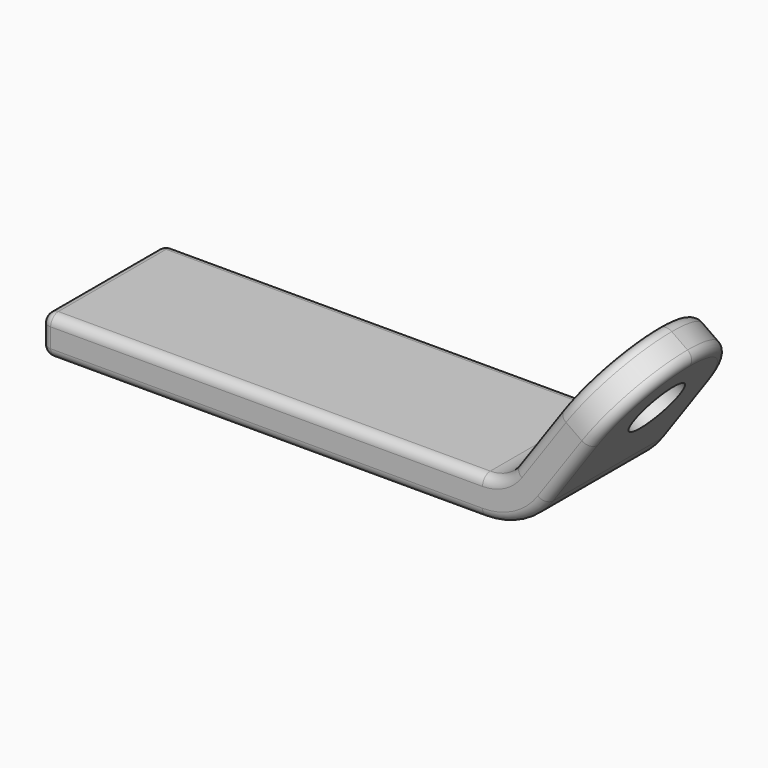
from build123d import *

# Parameters (mm, degrees)
F1_DEPTH     = 25.4
F2_R         = 9.525
F3_DEPTH     = 42.7816898715
F4_R         = 25.39999
F5_R         = 3.175
F6_W         = 5.0767767243
F6_H         = 5.0767767243
F7_DEPTH     = 3.175
F8_T1_DEPTH  = 142.613798458
F8_T3_DEPTH  = 25.40001
F8_T5_DEPTH  = 44.45
F8_T7_DEPTH  = 25.40001
F8_T9_DEPTH  = 2e-05
F8_T12_ANGLE = 90
F8_T14_ANGLE = 55
F8_T16_ANGLE = 55
F8_T18_ANGLE = 90
F8_T20_ANGLE = 90
F8_T22_ANGLE = 90
F8_T24_ANGLE = 55
F8_T26_ANGLE = 90
F8_T28_ANGLE = 90
F8_T30_ANGLE = 90
F8_T32_ANGLE = 55
F8_T34_ANGLE = 90


# Not quite as in the source:
# - a fillet or chamfer that OpenCascade refuses, or shapes differently, is made with other operations: its cross-section is extruded or revolved along the edge and cut away or added
# - a fillet or chamfer is up to 0.001 mm smaller than in the source, because OpenCascade refuses the exact size


with BuildPart() as f1:
    # F0 (on Front) → F1 (new body, symmetric)
    with BuildSketch(Plane.XZ):
        with BuildLine():
            Line((118.9895820573, 10.6313137069), (-26.7992164007, 10.6313137069))
            Line((-26.7992164007, 10.6313137069), (-26.7992164007, -2.0686862931))
            Line((-26.7992164007, -2.0686862931), (118.9895820573, -2.0686862931))
            ThreePointArc((118.9895820573, -2.0686862931), (130.7179968335, 0.8012385441), (139.7960439822, 8.7624722235))
            Line((139.7960439822, 8.7624722235), (168.9337269489, 50.3753960734))
            Line((168.9337269489, 50.3753960734), (158.5304959864, 57.6598168151))
            Line((158.5304959864, 57.6598168151), (129.3928130198, 16.0468929652))
            ThreePointArc((129.3928130198, 16.0468929652), (124.8537894454, 12.0662761255), (118.9895820573, 10.6313137069))
        make_face()
    extrude(amount=F1_DEPTH, both=True)

    # F2 (on face) → F3 (cut, through all)
    with BuildSketch(Plane(origin=(79.2843072841, 0, -55.515469622), x_dir=(0, -1, 0), z_dir=(-0.8191520443, 0, 0.5735764364))):
        with Locations((0, 115.9365137582)):
            Circle(F2_R)
    extrude(amount=-F3_DEPTH, mode=Mode.SUBTRACT)

    # F4 (radius 25.4 in the source; OpenCascade refuses exactly that, so slightly less here)
    f4_edges = [f1.edges().sort_by_distance(p)[0] for p in [
        (163.732111, 25.4, 54.017606),
        (163.732111, -25.4, 54.017606),
    ]]
    fillet(f4_edges, radius=F4_R)

    # F5
    f5_edges = [f1.edges().sort_by_distance(p)[0] for p in [
        (-26.799216, -25.4, 4.281314),
        (-26.799216, 25.4, 4.281314),
    ]]
    fillet(f5_edges, radius=F5_R)

    # F6 (on face) → F7 (cut)
    with BuildSketch(Plane(origin=(0, 0, -2.0686862931), x_dir=(1, 0, 0), z_dir=(0, 0, -1))):
        with Locations((4.9507835993, 0)):
            Rectangle(F6_W, F6_H)
    extrude(amount=-F7_DEPTH, mode=Mode.SUBTRACT)

    # F8: fillet of radius 3.175 on 24 edges, made by hand

    # F8_s2 → F8_t1 (cut)
    with BuildSketch(Plane.YZ.offset(-23.6242164007)):
        with BuildLine():
            ThreePointArc((25.4, 7.4563137069), (24.4700640303, 9.7013777371), (22.225, 10.6313137069))
            Line((22.225, 10.6313137069), (25.4, 10.6313137069))
            Line((25.4, 10.6313137069), (25.4, 7.4563137069))
        make_face()
        with BuildLine():
            ThreePointArc((-22.225, 10.6313137069), (-24.4700640303, 9.7013777371), (-25.4, 7.4563137069))
            Line((-25.4, 7.4563137069), (-25.4, 10.6313137069))
            Line((-25.4, 10.6313137069), (-22.225, 10.6313137069))
        make_face()
        with BuildLine():
            ThreePointArc((-22.225, -2.0686862931), (-24.4700640303, -1.1387503234), (-25.4, 1.1063137069))
            Line((-25.4, 1.1063137069), (-25.4, -2.0686862931))
            Line((-25.4, -2.0686862931), (-22.225, -2.0686862931))
        make_face()
        with BuildLine():
            ThreePointArc((25.4, 1.1063137069), (24.4700640303, -1.1387503234), (22.225, -2.0686862931))
            Line((22.225, -2.0686862931), (25.4, -2.0686862931))
            Line((25.4, -2.0686862931), (25.4, 1.1063137069))
        make_face()
    extrude(amount=F8_T1_DEPTH, mode=Mode.SUBTRACT)

    # F8_s4 → F8_t3 (cut)
    with BuildSketch(Plane(origin=(64.6773529548, 0, 92.3688327037), x_dir=(0, 1, 0), z_dir=(-0.5735764364, 0, -0.8191520443))):
        with BuildLine():
            ThreePointArc((25.4, 99.96326762), (24.4700640303, 97.7182035897), (22.225, 96.78826762))
            Line((22.225, 96.78826762), (25.4, 96.78826762))
            Line((25.4, 96.78826762), (25.4, 99.96326762))
        make_face()
        with BuildLine():
            ThreePointArc((-22.225, 96.78826762), (-24.4700640303, 97.7182035897), (-25.4, 99.96326762))
            Line((-25.4, 99.96326762), (-25.4, 96.78826762))
            Line((-25.4, 96.78826762), (-22.225, 96.78826762))
        make_face()
    extrude(amount=F8_T3_DEPTH, mode=Mode.SUBTRACT)

    # F8_s6 → F8_t5 (cut)
    with BuildSketch(Plane.XZ.offset(-22.225)):
        with BuildLine():
            ThreePointArc((-23.6242164007, 10.6313137069), (-25.869280431, 9.7013777371), (-26.7992164007, 7.4563137069))
            Line((-26.7992164007, 7.4563137069), (-26.7992164007, 10.6313137069))
            Line((-26.7992164007, 10.6313137069), (-23.6242164007, 10.6313137069))
        make_face()
        with BuildLine():
            ThreePointArc((-23.6242164007, -2.0686862931), (-25.869280431, -1.1387503234), (-26.7992164007, 1.1063137069))
            Line((-26.7992164007, 1.1063137069), (-26.7992164007, -2.0686862931))
            Line((-26.7992164007, -2.0686862931), (-23.6242164007, -2.0686862931))
        make_face()
    extrude(amount=F8_T5_DEPTH, mode=Mode.SUBTRACT)

    # F8_s8 → F8_t7 (cut)
    with BuildSketch(Plane(origin=(50.1085057357, 0, 71.5623625873), x_dir=(0, 1, 0), z_dir=(0.5735764364, 0, 0.8191520443))):
        with BuildLine():
            ThreePointArc((25.4, -106.31326762), (24.4700640303, -108.5583316502), (22.225, -109.48826762))
            Line((22.225, -109.48826762), (25.4, -109.48826762))
            Line((25.4, -109.48826762), (25.4, -106.31326762))
        make_face()
        with BuildLine():
            ThreePointArc((-22.225, -109.48826762), (-24.4700640303, -108.5583316502), (-25.4, -106.31326762))
            Line((-25.4, -106.31326762), (-25.4, -109.48826762))
            Line((-25.4, -109.48826762), (-22.225, -109.48826762))
        make_face()
    extrude(amount=F8_T7_DEPTH, mode=Mode.SUBTRACT)

    # F8_s10 → F8_t9 (cut)
    with BuildSketch(Plane.XZ.offset(-1e-05)):
        with BuildLine():
            ThreePointArc((167.1126217635, 47.7745883328), (167.6385786386, 50.1470264823), (166.3329192083, 52.1965012588))
            Line((166.3329192083, 52.1965012588), (168.9337269489, 50.3753960734))
            Line((168.9337269489, 50.3753960734), (167.1126217635, 47.7745883328))
        make_face()
        with BuildLine():
            ThreePointArc((156.709390801, 55.0590090745), (158.7588655775, 56.3646685049), (161.131303727, 55.8387116297))
            Line((161.131303727, 55.8387116297), (158.5304959864, 57.6598168151))
            Line((158.5304959864, 57.6598168151), (156.709390801, 55.0590090745))
        make_face()
    extrude(amount=F8_T9_DEPTH, mode=Mode.SUBTRACT)

    # F8_s11 → F8_t12 (revolve, cut)
    with BuildSketch(Plane(origin=(64.6773529548, 0, 92.3688327037), x_dir=(0, 1, 0), z_dir=(-0.5735764364, 0, -0.8191520443))):
        with BuildLine():
            ThreePointArc((25.4, 99.96326762), (24.4700640303, 97.7182035897), (22.225, 96.78826762))
            Line((22.225, 96.78826762), (25.4, 96.78826762))
            Line((25.4, 96.78826762), (25.4, 99.96326762))
        make_face()
    revolve(axis=Axis((143.9616602388, 1e-05, 36.8533630817), (0.8191520443, 0, -0.5735764364)), revolution_arc=F8_T12_ANGLE, mode=Mode.SUBTRACT)

    # F8_s13 → F8_t14 (revolve, cut)
    with BuildSketch(Plane.YZ.offset(118.9895820573)):
        with BuildLine():
            ThreePointArc((25.4, 1.1063137069), (24.4700640303, -1.1387503234), (22.225, -2.0686862931))
            Line((22.225, -2.0686862931), (25.4, -2.0686862931))
            Line((25.4, -2.0686862931), (25.4, 1.1063137069))
        make_face()
    revolve(axis=Axis((118.9895820573, 25.4, 23.3313137069), (0, -1, 0)), revolution_arc=F8_T14_ANGLE, mode=Mode.SUBTRACT)

    # F8_s15 → F8_t16 (revolve, cut)
    with BuildSketch(Plane(origin=(50.1085057357, 0, 71.5623625873), x_dir=(0, 1, 0), z_dir=(0.5735764364, 0, 0.8191520443))):
        with BuildLine():
            ThreePointArc((25.4, -99.96326762), (24.4700640303, -97.7182035897), (22.225, -96.78826762))
            Line((22.225, -96.78826762), (25.4, -96.78826762))
            Line((25.4, -96.78826762), (25.4, -99.96326762))
        make_face()
    revolve(axis=Axis((118.9895820573, 25.4, 23.3313137069), (0, 1, 0)), revolution_arc=F8_T16_ANGLE, mode=Mode.SUBTRACT)

    # F8_s17 → F8_t18 (revolve, cut)
    with BuildSketch(Plane.YZ.offset(-23.6242164007)):
        with BuildLine():
            ThreePointArc((22.225, -2.0686862931), (24.4700640303, -1.1387503234), (25.4, 1.1063137069))
            Line((25.4, 1.1063137069), (25.4, -2.0686862931))
            Line((25.4, -2.0686862931), (22.225, -2.0686862931))
        make_face()
    revolve(axis=Axis((-23.6242164007, 22.225, -2.0686862931), (0, 0, 1)), revolution_arc=F8_T18_ANGLE, mode=Mode.SUBTRACT)

    # F8_s19 → F8_t20 (revolve, cut)
    with BuildSketch(Plane.YZ.offset(-23.6242164007)):
        with BuildLine():
            ThreePointArc((-22.225, -2.0686862931), (-24.4700640303, -1.1387503234), (-25.4, 1.1063137069))
            Line((-25.4, 1.1063137069), (-25.4, -2.0686862931))
            Line((-25.4, -2.0686862931), (-22.225, -2.0686862931))
        make_face()
    revolve(axis=Axis((-23.6242164007, -22.225, -2.0686862931), (0, 0, -1)), revolution_arc=F8_T20_ANGLE, mode=Mode.SUBTRACT)

    # F8_s21 → F8_t22 (revolve, cut)
    with BuildSketch(Plane.YZ.offset(-23.6242164007)):
        with BuildLine():
            ThreePointArc((25.4, 7.4563137069), (24.4700640303, 9.7013777371), (22.225, 10.6313137069))
            Line((22.225, 10.6313137069), (25.4, 10.6313137069))
            Line((25.4, 10.6313137069), (25.4, 7.4563137069))
        make_face()
    revolve(axis=Axis((-23.6242164007, 22.225, 10.6313137069), (0, 0, 1)), revolution_arc=F8_T22_ANGLE, mode=Mode.SUBTRACT)

    # F8_s23 → F8_t24 (revolve, cut)
    with BuildSketch(Plane.YZ.offset(118.9895820573)):
        with BuildLine():
            ThreePointArc((-22.225, -2.0686862931), (-24.4700640303, -1.1387503234), (-25.4, 1.1063137069))
            Line((-25.4, 1.1063137069), (-25.4, -2.0686862931))
            Line((-25.4, -2.0686862931), (-22.225, -2.0686862931))
        make_face()
    revolve(axis=Axis((118.9895820573, -25.4, 23.3313137069), (0, -1, 0)), revolution_arc=F8_T24_ANGLE, mode=Mode.SUBTRACT)

    # F8_s25 → F8_t26 (revolve, cut)
    with BuildSketch(Plane.YZ.offset(-23.6242164007)):
        with BuildLine():
            ThreePointArc((-22.225, 10.6313137069), (-24.4700640303, 9.7013777371), (-25.4, 7.4563137069))
            Line((-25.4, 7.4563137069), (-25.4, 10.6313137069))
            Line((-25.4, 10.6313137069), (-22.225, 10.6313137069))
        make_face()
    revolve(axis=Axis((-23.6242164007, -22.225, 10.6313137069), (0, 0, -1)), revolution_arc=F8_T26_ANGLE, mode=Mode.SUBTRACT)

    # F8_s27 → F8_t28 (revolve, cut)
    with BuildSketch(Plane(origin=(64.6773529548, 0, 92.3688327037), x_dir=(0, 1, 0), z_dir=(-0.5735764364, 0, -0.8191520443))):
        with BuildLine():
            ThreePointArc((22.225, 109.48826762), (24.4700640303, 108.5583316502), (25.4, 106.31326762))
            Line((25.4, 106.31326762), (25.4, 109.48826762))
            Line((25.4, 109.48826762), (22.225, 109.48826762))
        make_face()
    revolve(axis=Axis((154.3648912013, 1e-05, 29.56894234), (0.8191520443, 0, -0.5735764364)), revolution_arc=F8_T28_ANGLE, mode=Mode.SUBTRACT)

    # F8_s29 → F8_t30 (revolve, cut)
    with BuildSketch(Plane.XZ.offset(1e-05)):
        with BuildLine():
            ThreePointArc((167.1126217635, 47.7745883328), (167.6385786386, 50.1470264823), (166.3329192083, 52.1965012588))
            Line((166.3329192083, 52.1965012588), (168.9337269489, 50.3753960734))
            Line((168.9337269489, 50.3753960734), (167.1126217635, 47.7745883328))
        make_face()
    revolve(axis=Axis((154.3648912013, -1e-05, 29.56894234), (0.8191520443, 0, -0.5735764364)), revolution_arc=F8_T30_ANGLE, mode=Mode.SUBTRACT)

    # F8_s31 → F8_t32 (revolve, cut)
    with BuildSketch(Plane(origin=(50.1085057357, 0, 71.5623625873), x_dir=(0, 1, 0), z_dir=(0.5735764364, 0, 0.8191520443))):
        with BuildLine():
            ThreePointArc((-22.225, -96.78826762), (-24.4700640303, -97.7182035897), (-25.4, -99.96326762))
            Line((-25.4, -99.96326762), (-25.4, -96.78826762))
            Line((-25.4, -96.78826762), (-22.225, -96.78826762))
        make_face()
    revolve(axis=Axis((118.9895820573, -25.4, 23.3313137069), (0, 1, 0)), revolution_arc=F8_T32_ANGLE, mode=Mode.SUBTRACT)

    # F8_s33 → F8_t34 (revolve, cut)
    with BuildSketch(Plane.XZ.offset(1e-05)):
        with BuildLine():
            ThreePointArc((156.709390801, 55.0590090745), (158.7588655775, 56.3646685049), (161.131303727, 55.8387116297))
            Line((161.131303727, 55.8387116297), (158.5304959864, 57.6598168151))
            Line((158.5304959864, 57.6598168151), (156.709390801, 55.0590090745))
        make_face()
    revolve(axis=Axis((143.9616602388, -1e-05, 36.8533630817), (0.8191520443, 0, -0.5735764364)), revolution_arc=F8_T34_ANGLE, mode=Mode.SUBTRACT)


solid = f1.part
